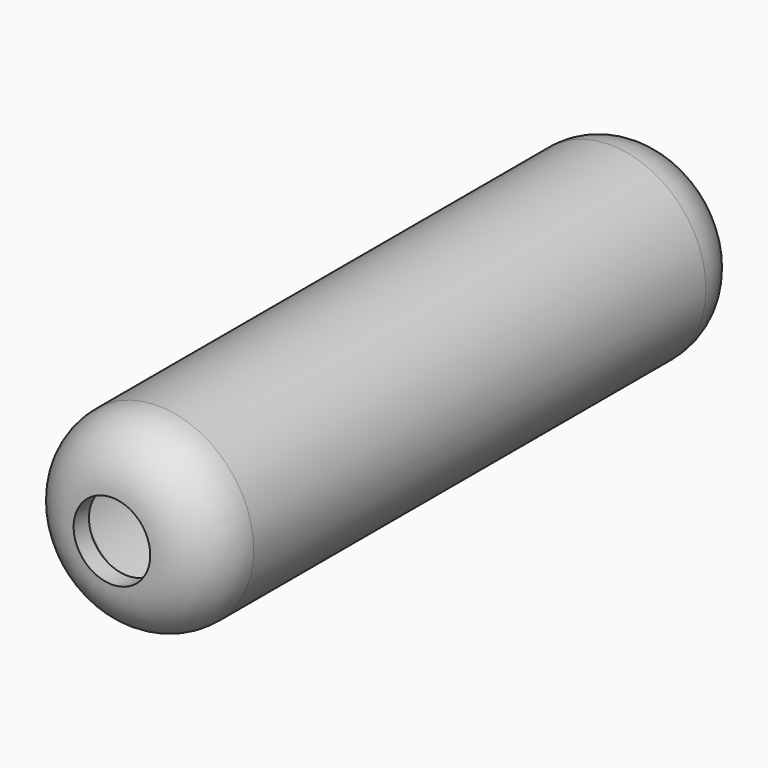
from build123d import *

# Parameters (mm, degrees)
F0_R     = 12.7
F1_DEPTH = 90.17
F2_R     = 7.62
F3_T     = -2.54


# Not quite as in the source:
# - a shell that OpenCascade refuses in one call is made with other operations: the cavity is built on its own and cut out


with BuildPart() as f1:
    # F0 (on Front) → F1 (new body)
    with BuildSketch(Plane.XZ):
        Circle(F0_R)
    extrude(amount=F1_DEPTH)

    # F2
    f2_edges = [f1.edges().sort_by_distance(p)[0] for p in [
        (-12.7, -90.17, 0),
        (-12.7, 0, 0),
    ]]
    fillet(f2_edges, radius=F2_R)

    # F3: a shell. OpenCascade refuses it in one call, so the cavity is built on its own and cut out:
    # the body offset inwards by the wall thickness, plus a prism from it out through each open face.
    f3_core = offset(f1.part, amount=F3_T, mode=Mode.PRIVATE)
    f3_exits = [f3_core.faces().sort_by_distance(p)[0] for p in [
        (0, -87.63, 0),
    ]]
    add(f3_core, mode=Mode.SUBTRACT)
    extrude(f3_exits, amount=-F3_T, mode=Mode.SUBTRACT)


solid = f1.part
